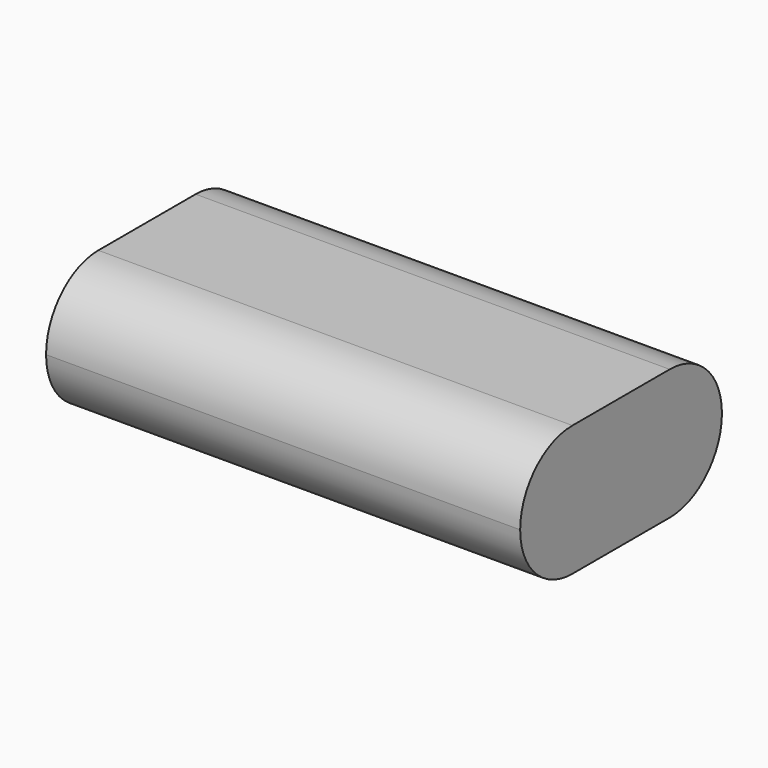
from build123d import *

# Parameters (mm, degrees)
F1_W     = 69
F1_H     = 36.7
F2_DEPTH = 19
F3_R     = 9.49999


# Not quite as in the source:
# - a fillet or chamfer is up to 0.001 mm smaller than in the source, because OpenCascade refuses the exact size


with BuildPart() as f2:
    # F1 (on Top) → F2 (new body)
    with BuildSketch(Plane.XY):
        with Locations((1.7897747457, -8.3416857903)):
            Rectangle(F1_W, F1_H)
    extrude(amount=F2_DEPTH)

    # F3 (radius 9.5 in the source; OpenCascade refuses exactly that, so slightly less here)
    f3_edges = [f2.edges().sort_by_distance(p)[0] for p in [
        (1.789775, -26.691686, 19),
        (1.789775, -26.691686, 0),
        (1.789775, 10.008314, 19),
        (1.789775, 10.008314, 0),
    ]]
    fillet(f3_edges, radius=F3_R)


solid = f2.part
